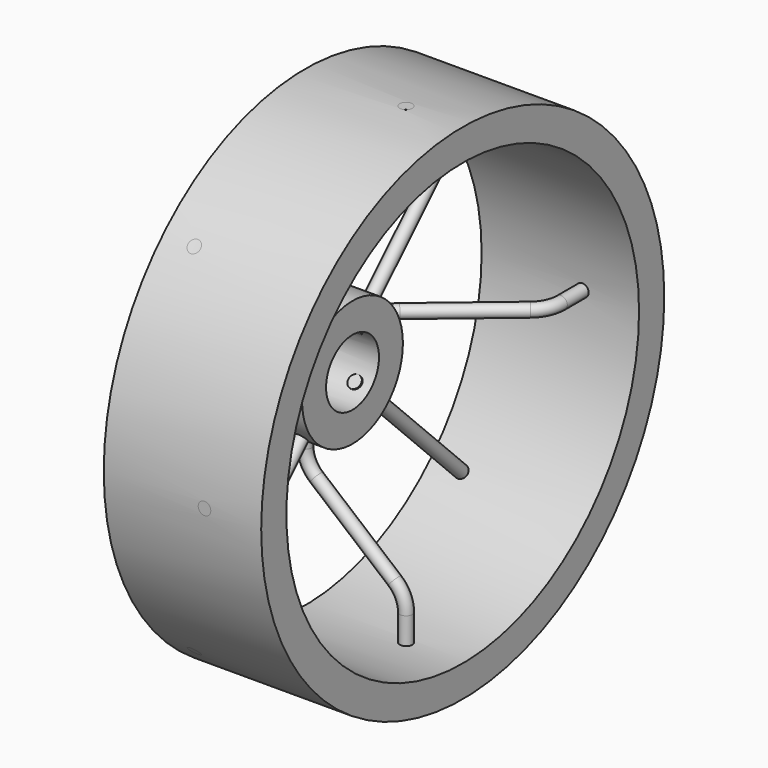
from build123d import *

# Parameters (mm, degrees)
F3_R      = 1
F0_R      = 10
F0_R_2    = 5.25
F5_DEPTH  = 7.5
F0_R_3    = 40
F0_R_4    = 35
F6_DEPTH  = 25
F7_COUNT  = 4
F11_R     = 1
F12_REACH = 54.3979697611
F13_COUNT = 4


with BuildPart() as f4:
    # F4: sweep along a path in F1
    with BuildLine(Plane.XZ) as f4_path:
        Line((0, 5), (0, 12.6684617092))
        ThreePointArc((0, 12.6684617092), (0.4684610648, 14.7815530179), (1.7860619516, 16.4986839248))
        Line((1.7860619516, 16.4986839248), (14.2139380484, 26.926910174))
        ThreePointArc((14.2139380484, 26.926910174), (15.5315389352, 28.6440410809), (16, 30.7571323896))
        Line((16, 30.7571323896), (16, 40))
    # F3 (on plane+point) → F4 (sweep)
    with BuildSketch(Plane.XY.offset(5)):
        Circle(F3_R)
    sweep(path=f4_path.line)


with BuildPart() as f5:
    # F0 (on Right) → F5 (new body, symmetric)
    with BuildSketch(Plane.YZ):
        Circle(F0_R)
        Circle(F0_R_2, mode=Mode.SUBTRACT)
    extrude(amount=F5_DEPTH, both=True)


with BuildPart() as f6:
    # F0 (on Right) → F6 (new body)
    with BuildSketch(Plane.YZ):
        Circle(F0_R_3)
        Circle(F0_R_4, mode=Mode.SUBTRACT)
    extrude(amount=F6_DEPTH)


with BuildPart() as f7_1:
    # F7: instance of F4
    add(f4.part.rotate(Axis((0, 0, 0), (1, 0, 0)), 1 * 360 / F7_COUNT))


with BuildPart() as f7_2:
    # F7: instance of F4
    add(f4.part.rotate(Axis((0, 0, 0), (1, 0, 0)), 2 * 360 / F7_COUNT))


with BuildPart() as f7_3:
    # F7: instance of F4
    add(f4.part.rotate(Axis((0, 0, 0), (1, 0, 0)), 3 * 360 / F7_COUNT))


with BuildPart() as f6_1:
    add(f6.part)

    # F8: cut F4, F7_1, F7_2, F7_3
    add(f4.part, mode=Mode.SUBTRACT)
    add(f7_1.part, mode=Mode.SUBTRACT)
    add(f7_2.part, mode=Mode.SUBTRACT)
    add(f7_3.part, mode=Mode.SUBTRACT)


with BuildPart() as f5_1:
    add(f5.part)

    # F8: cut F4, F7_1, F7_2, F7_3
    add(f4.part, mode=Mode.SUBTRACT)
    add(f7_1.part, mode=Mode.SUBTRACT)
    add(f7_2.part, mode=Mode.SUBTRACT)
    add(f7_3.part, mode=Mode.SUBTRACT)


with BuildPart() as f12:
    f12_end = f6_1.part.faces().sort_by_distance((12.5, -40, 0))[0]
    # F11 (on face) → F12 (new body, up to a face of F6 that its end follows)
    with BuildSketch(Plane(origin=(0, 3.5355339059, 3.5355339059), x_dir=(-1, 0, 0), z_dir=(0, 0.7071067812, 0.7071067812))):
        with Locations((-5, 0)):
            Circle(F11_R)
    f12_long = extrude(amount=F12_REACH, mode=Mode.PRIVATE)
    add(split(f12_long, bisect_by=f12_end, keep=Keep.BOTTOM, mode=Mode.PRIVATE))


with BuildPart() as f13_1:
    # F13: instance of F12
    add(f12.part.rotate(Axis((-7.5, 0, 0), (1, 0, 0)), 1 * 360 / F13_COUNT))


with BuildPart() as f13_2:
    # F13: instance of F12
    add(f12.part.rotate(Axis((-7.5, 0, 0), (1, 0, 0)), 2 * 360 / F13_COUNT))


with BuildPart() as f13_3:
    # F13: instance of F12
    add(f12.part.rotate(Axis((-7.5, 0, 0), (1, 0, 0)), 3 * 360 / F13_COUNT))


with BuildPart() as f6_2:
    add(f6_1.part)

    # F14: cut F13_3, F12, F13_1, F13_2
    add(f13_3.part, mode=Mode.SUBTRACT)
    add(f12.part, mode=Mode.SUBTRACT)
    add(f13_1.part, mode=Mode.SUBTRACT)
    add(f13_2.part, mode=Mode.SUBTRACT)


with BuildPart() as f5_2:
    add(f5_1.part)

    # F14: cut F13_3, F12, F13_1, F13_2
    add(f13_3.part, mode=Mode.SUBTRACT)
    add(f12.part, mode=Mode.SUBTRACT)
    add(f13_1.part, mode=Mode.SUBTRACT)
    add(f13_2.part, mode=Mode.SUBTRACT)


solid = Compound([f4.part, f7_1.part, f7_2.part, f7_3.part, f12.part, f13_1.part, f13_2.part, f13_3.part, f6_2.part, f5_2.part])
